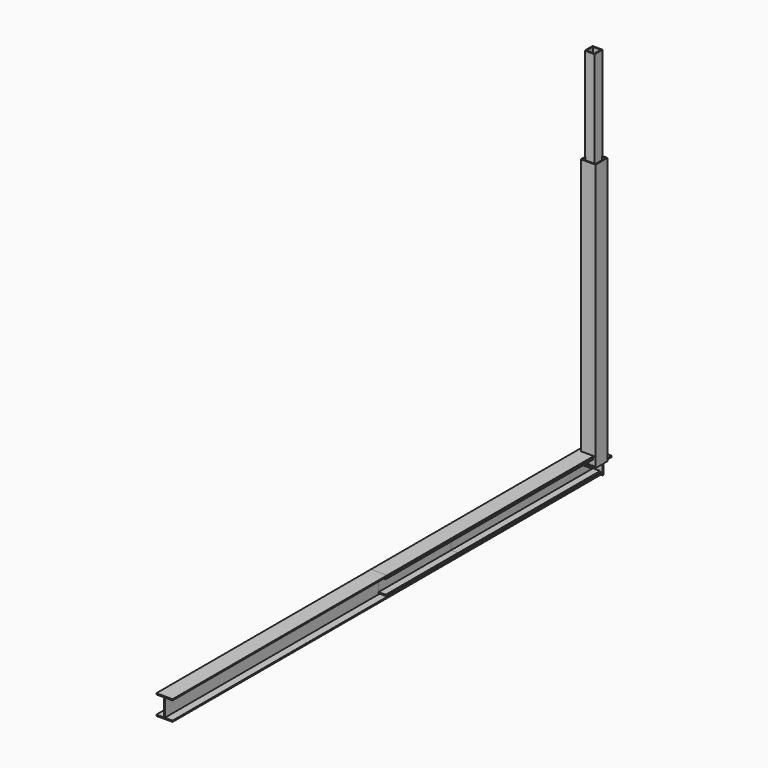
from build123d import *

# Parameters (mm, degrees)
F3_DEPTH  = 5486.4
F4_DEPTH  = 2743.2
F6_DEPTH  = 2754.7316
F7_DEPTH  = 1828.8
F8_W      = 82.55
F8_H      = 82.55
F9_DEPTH  = 1219.2
F10_W     = 133.35
F10_H     = 133.35
F11_DEPTH = 1828.8
F12_DEPTH = 3688.8928
F13_W     = 166.0144
F13_H     = 254
F13_R     = 7.9375
F14_DEPTH = 12.7
F15_W     = 152.4
F15_H     = 152.4
F15_R     = 4.7625
F16_DEPTH = 12.7
F17_W     = 154.432
F17_H     = 254
F17_R     = 7.9375
F18_DEPTH = 12.7
F19_W     = 203.2
F19_H     = 203.2
F19_R     = 6.35
F20_DEPTH = 12.7
F21_DEPTH = 2731.3636


# Not quite as in the source:
# - a variable given as a bare number and used for a length is read in inches; the dataset says mm whatever the document's units were


with BuildPart() as f3:
    # F2 (on Front) → F3 (new body)
    with BuildSketch(Plane.XZ):
        Polygon((-3.6195, 90.551), (-3.6195, 0), (-3.6195, -90.551), (-82.9945, -90.551), (-82.9945, -102.362), (0, -102.362), (82.9945, -102.362), (82.9945, -90.551), (3.6195, -90.551), (3.6195, 0), (3.6195, 90.551), (82.9945, 90.551), (82.9945, 102.362), (0, 102.362), (-82.9945, 102.362), (-82.9945, 90.551), align=None)
    extrude(amount=F3_DEPTH)


with BuildPart() as f4:
    # F2 (on Front) → F4 (new body)
    with BuildSketch(Plane.XZ):
        Polygon((-3.6195, 90.551), (-3.6195, 0), (-3.6195, -90.551), (-82.9945, -90.551), (-82.9945, -102.362), (0, -102.362), (82.9945, -102.362), (82.9945, -90.551), (3.6195, -90.551), (3.6195, 0), (3.6195, 90.551), (82.9945, 90.551), (82.9945, 102.362), (0, 102.362), (-82.9945, 102.362), (-82.9945, 90.551), align=None)
    extrude(amount=F4_DEPTH)


with BuildPart() as f6:
    # F5 (on Front) → F6 (new body)
    with BuildSketch(Plane.XZ):
        Polygon((-4.064, 69.469), (-4.064, 0), (-4.064, -69.469), (-77.216, -69.469), (-77.216, -81.026), (0, -81.026), (77.216, -81.026), (77.216, -69.469), (4.064, -69.469), (4.064, 0), (4.064, 69.469), (77.216, 69.469), (77.216, 81.026), (0, 81.026), (-77.216, 81.026), (-77.216, 69.469), align=None)
    extrude(amount=F6_DEPTH)


with BuildPart() as f7:
    # F5 (on Front) → F7 (new body)
    with BuildSketch(Plane.XZ):
        Polygon((-4.064, 69.469), (-4.064, 0), (-4.064, -69.469), (-77.216, -69.469), (-77.216, -81.026), (0, -81.026), (77.216, -81.026), (77.216, -69.469), (4.064, -69.469), (4.064, 0), (4.064, 69.469), (77.216, 69.469), (77.216, 81.026), (0, 81.026), (-77.216, 81.026), (-77.216, 69.469), align=None)
    extrude(amount=F7_DEPTH)


with BuildPart() as f9:
    # F8 (on Top) → F9 (new body)
    with BuildSketch(Plane.XY):
        with BuildLine():
            Line((-47.625, -50.8), (47.625, -50.8))
            ThreePointArc((47.625, -50.8), (49.8700640303, -49.8700640303), (50.8, -47.625))
            Line((50.8, -47.625), (50.8, 47.625))
            ThreePointArc((50.8, 47.625), (49.8700640303, 49.8700640303), (47.625, 50.8))
            Line((47.625, 50.8), (-47.625, 50.8))
            ThreePointArc((-47.625, 50.8), (-49.8700640303, 49.8700640303), (-50.8, 47.625))
            Line((-50.8, 47.625), (-50.8, -47.625))
            ThreePointArc((-50.8, -47.625), (-49.8700640303, -49.8700640303), (-47.625, -50.8))
        make_face()
        Rectangle(F8_W, F8_H, mode=Mode.SUBTRACT)
    extrude(amount=F9_DEPTH)


with BuildPart() as f11:
    # F10 (on Top) → F11 (new body)
    with BuildSketch(Plane.XY):
        with BuildLine():
            Line((-47.625, -101.6), (98.425, -101.6))
            ThreePointArc((98.425, -101.6), (100.6700640303, -100.6700640303), (101.6, -98.425))
            Line((101.6, -98.425), (101.6, 47.625))
            ThreePointArc((101.6, 47.625), (100.6700640303, 49.8700640303), (98.425, 50.8))
            Line((98.425, 50.8), (-47.625, 50.8))
            ThreePointArc((-47.625, 50.8), (-49.8700640303, 49.8700640303), (-50.8, 47.625))
            Line((-50.8, 47.625), (-50.8, -98.425))
            ThreePointArc((-50.8, -98.425), (-49.8700640303, -100.6700640303), (-47.625, -101.6))
        make_face()
        with Locations((25.4, -25.4)):
            Rectangle(F10_W, F10_H, mode=Mode.SUBTRACT)
    extrude(amount=F11_DEPTH)


with BuildPart() as f12:
    # F8 (on Top) → F12 (new body)
    with BuildSketch(Plane.XY):
        with BuildLine():
            Line((-47.625, -50.8), (47.625, -50.8))
            ThreePointArc((47.625, -50.8), (49.8700640303, -49.8700640303), (50.8, -47.625))
            Line((50.8, -47.625), (50.8, 47.625))
            ThreePointArc((50.8, 47.625), (49.8700640303, 49.8700640303), (47.625, 50.8))
            Line((47.625, 50.8), (-47.625, 50.8))
            ThreePointArc((-47.625, 50.8), (-49.8700640303, 49.8700640303), (-50.8, 47.625))
            Line((-50.8, 47.625), (-50.8, -47.625))
            ThreePointArc((-50.8, -47.625), (-49.8700640303, -49.8700640303), (-47.625, -50.8))
        make_face()
        Rectangle(F8_W, F8_H, mode=Mode.SUBTRACT)
    extrude(amount=F12_DEPTH)


with BuildPart() as f14:
    # F13 (on Top) → F14 (new body)
    with BuildSketch(Plane.XY):
        Rectangle(F13_W, F13_H)
        with Locations((-57.6072, -101.6)):
            Circle(F13_R, mode=Mode.SUBTRACT)
        with Locations((57.6072, -101.6)):
            Circle(F13_R, mode=Mode.SUBTRACT)
        with Locations((-57.6072, 101.6)):
            Circle(F13_R, mode=Mode.SUBTRACT)
        with Locations((57.6072, 101.6)):
            Circle(F13_R, mode=Mode.SUBTRACT)
    extrude(amount=F14_DEPTH)


with BuildPart() as f16:
    # F15 (on Top) → F16 (new body)
    with BuildSketch(Plane.XY):
        Rectangle(F15_W, F15_H)
        with Locations((-63.5, -63.5)):
            Circle(F15_R, mode=Mode.SUBTRACT)
        with Locations((63.5, -63.5)):
            Circle(F15_R, mode=Mode.SUBTRACT)
        with Locations((-63.5, 63.5)):
            Circle(F15_R, mode=Mode.SUBTRACT)
        with Locations((63.5, 63.5)):
            Circle(F15_R, mode=Mode.SUBTRACT)
    extrude(amount=F16_DEPTH)


with BuildPart() as f18:
    # F17 (on Top) → F18 (new body)
    with BuildSketch(Plane.XY):
        Rectangle(F17_W, F17_H)
        with Locations((-51.816, -101.6)):
            Circle(F17_R, mode=Mode.SUBTRACT)
        with Locations((51.816, -101.6)):
            Circle(F17_R, mode=Mode.SUBTRACT)
        with Locations((-51.816, 101.6)):
            Circle(F17_R, mode=Mode.SUBTRACT)
        with Locations((51.816, 101.6)):
            Circle(F17_R, mode=Mode.SUBTRACT)
    extrude(amount=F18_DEPTH)


with BuildPart() as f20:
    # F19 (on Front) → F20 (new body)
    with BuildSketch(Plane.XZ):
        Rectangle(F19_W, F19_H)
        with Locations((-80.9625, -80.9625)):
            Circle(F19_R, mode=Mode.SUBTRACT)
        with Locations((80.9625, -80.9625)):
            Circle(F19_R, mode=Mode.SUBTRACT)
        with Locations((-80.9625, 80.9625)):
            Circle(F19_R, mode=Mode.SUBTRACT)
        with Locations((80.9625, 80.9625)):
            Circle(F19_R, mode=Mode.SUBTRACT)
    extrude(amount=F20_DEPTH)


with BuildPart() as f21:
    # F10 (on Top) → F21 (new body)
    with BuildSketch(Plane.XY):
        with BuildLine():
            Line((-47.625, -101.6), (98.425, -101.6))
            ThreePointArc((98.425, -101.6), (100.6700640303, -100.6700640303), (101.6, -98.425))
            Line((101.6, -98.425), (101.6, 47.625))
            ThreePointArc((101.6, 47.625), (100.6700640303, 49.8700640303), (98.425, 50.8))
            Line((98.425, 50.8), (-47.625, 50.8))
            ThreePointArc((-47.625, 50.8), (-49.8700640303, 49.8700640303), (-50.8, 47.625))
            Line((-50.8, 47.625), (-50.8, -98.425))
            ThreePointArc((-50.8, -98.425), (-49.8700640303, -100.6700640303), (-47.625, -101.6))
        make_face()
        with Locations((25.4, -25.4)):
            Rectangle(F10_W, F10_H, mode=Mode.SUBTRACT)
    extrude(amount=F21_DEPTH)


solid = Compound([f3.part, f4.part, f6.part, f7.part, f9.part, f11.part, f12.part, f14.part, f16.part, f18.part, f20.part, f21.part])
